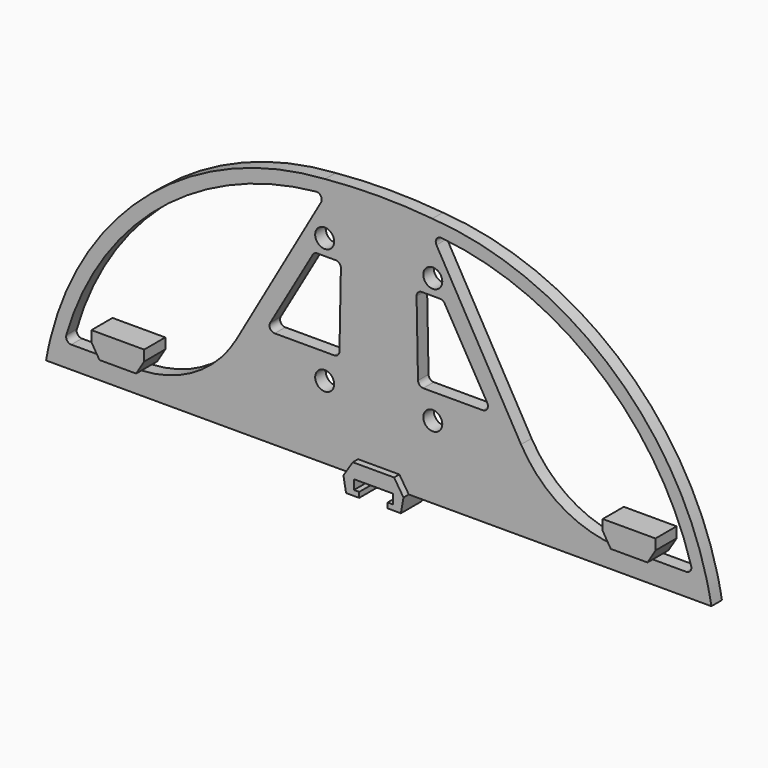
from build123d import *

# Parameters (mm, degrees)
F0_R     = 18
F1_DEPTH = 12.5
F2_R     = 10
F3_DEPTH = 25


# Not quite as in the source:
# - a feature names something its author has since deleted; it is built from what else it names


with BuildPart() as f1:
    # F0 (on Front) → F1 (new body, symmetric)
    with BuildSketch(Plane.XZ):
        with BuildLine():
            Line((56.9371554598, -75), (595.9911190147, -75))
            Line((595.9911190147, -75), (595.9911190147, -33))
            Line((595.9911190147, -33), (519.5849960263, -33))
            Line((519.5849960263, -33), (450, -33))
            ThreePointArc((450, -33), (345.7777045638, -0.7457623443), (269.8662378191, 77.6128487294))
            Line((269.8662378191, 77.6128487294), (100, 375))
            Line((100, 375), (0, 375))
            Line((0, 375), (-100, 375))
            Line((-100, 375), (-269.8662378191, 77.6128487294))
            ThreePointArc((-269.8662378191, 77.6128487294), (-345.7777045638, -0.7457623443), (-450, -33))
            Line((-450, -33), (-484.7924980132, -33))
            Line((-484.7924980132, -33), (-519.5849960263, -33))
            Line((-519.5849960263, -33), (-595.9911190147, -33))
            Line((-595.9911190147, -33), (-595.9911190147, -75))
            Line((-595.9911190147, -75), (-56.9371554598, -75))
            Line((-56.9371554598, -75), (-39.1645557923, -47.3871512706))
            Line((-39.1645557923, -47.3871512706), (3.3388429378, -47.3871512706))
            Line((3.3388429378, -47.3871512706), (39.1645557923, -47.3871512706))
            Line((39.1645557923, -47.3871512706), (56.9371554598, -75))
        make_face()
        with Locations((-102.5, 63)):
            Circle(F0_R, mode=Mode.SUBTRACT)
        with Locations((102.5, 63)):
            Circle(F0_R, mode=Mode.SUBTRACT)
        with BuildLine():
            ThreePointArc((-74.4771999255, 121.0282629209), (-77.4732139948, 114.0830094681), (-84.4753157308, 111.2223771768))
            Line((-84.4753157308, 111.2223771768), (-197.1059338565, 111.2223771768))
            ThreePointArc((-197.1059338565, 111.2223771768), (-205.7661878943, 116.2223771768), (-205.7661878943, 126.2223771768))
            Line((-205.7661878943, 126.2223771768), (-125.0655397306, 266))
            ThreePointArc((-125.0655397306, 266), (-121.4052856928, 269.6602540378), (-116.4052856928, 271))
            Line((-116.4052856928, 271), (-81.7615214746, 271))
            ThreePointArc((-81.7615214746, 271), (-74.622153766, 268.0021017359), (-71.7634056693, 260.8058857441))
            Line((-71.7634056693, 260.8058857441), (-74.4771999255, 121.0282629209))
        make_face(mode=Mode.SUBTRACT)
        with Locations((-102.5, 301)):
            Circle(F0_R, mode=Mode.SUBTRACT)
        with BuildLine():
            ThreePointArc((84.4753157308, 111.2223771768), (77.4732139948, 114.0830094681), (74.4771999255, 121.0282629209))
            Line((74.4771999255, 121.0282629209), (71.7634056693, 260.8058857441))
            ThreePointArc((71.7634056693, 260.8058857441), (74.622153766, 268.0021017359), (81.7615214746, 271))
            Line((81.7615214746, 271), (116.4052856928, 271))
            ThreePointArc((116.4052856928, 271), (121.4052856928, 269.6602540378), (125.0655397306, 266))
            Line((125.0655397306, 266), (205.7661878943, 126.2223771768))
            ThreePointArc((205.7661878943, 126.2223771768), (205.7661878943, 116.2223771768), (197.1059338565, 111.2223771768))
            Line((197.1059338565, 111.2223771768), (84.4753157308, 111.2223771768))
        make_face(mode=Mode.SUBTRACT)
        with Locations((102.5, 301)):
            Circle(F0_R, mode=Mode.SUBTRACT)
        with BuildLine():
            ThreePointArc((100, 375), (413.732568712, 250.914148912), (595.9911190147, -33))
            Line((595.9911190147, -33), (621.814123166, -33))
            ThreePointArc((621.814123166, -33), (432.1619331745, 268.1134366241), (101.6213617791, 399.9473683177))
            ThreePointArc((101.6213617791, 399.9473683177), (0, 404.6514727579), (-101.6213617791, 399.9473683177))
            ThreePointArc((-101.6213617791, 399.9473683177), (-432.1619331745, 268.1134366241), (-621.814123166, -33))
            Line((-621.814123166, -33), (-595.9911190147, -33))
            ThreePointArc((-595.9911190147, -33), (-413.732568712, 250.914148912), (-100, 375))
            Line((-100, 375), (0, 375))
            Line((0, 375), (100, 375))
        make_face()
        with BuildLine():
            Line((-595.9911190147, -75), (-595.9911190147, -33))
            Line((-595.9911190147, -33), (-621.814123166, -33))
            ThreePointArc((-621.814123166, -33), (-626.6847460238, -53.9163527136), (-630.7708927375, -75))
            Line((-630.7708927375, -75), (-595.9911190147, -75))
        make_face()
        with BuildLine():
            Line((595.9911190147, -33), (595.9911190147, -75))
            Line((595.9911190147, -75), (630.7708927375, -75))
            ThreePointArc((630.7708927375, -75), (626.6847460238, -53.9163527136), (621.814123166, -33))
            Line((621.814123166, -33), (595.9911190147, -33))
        make_face()
    extrude(amount=F1_DEPTH, both=True)

    # F2
    f2_edges = [f1.edges().sort_by_distance(p)[0] for p in [
        (-100, 0, 375),
        (100, 0, 375),
        (595.991119, 0, -33),
        (-595.991119, 0, -33),
    ]]
    fillet(f2_edges, radius=F2_R)

    # F0 (on Front) → F3 (join, symmetric)
    with BuildSketch(Plane.XZ):
        Polygon((-484.7924980132, -33), (-450, -33), (-434.7924980132, -8), (-434.7924980132, 12), (-484.7924980132, 12), (-534.7924980132, 12), (-534.7924980132, -8), (-519.5849960263, -33), align=None)
        Polygon((37, -75), (56.9371554598, -75), (39.1645557923, -47.3871512706), (3.3388429378, -47.3871512706), (-39.1645557923, -47.3871512706), (-56.9371554598, -75), (-37, -75), (0, -75), align=None)
        Polygon((52, -103), (56.9371554598, -75), (37, -75), (37, -93), (27, -93), (27, -103), align=None)
        Polygon((-37, -93), (-37, -75), (-56.9371554598, -75), (-52, -103), (-27, -103), (-27, -93), align=None)
        Polygon((450, -33), (519.5849960263, -33), (534.7924980132, -8), (534.7924980132, 12), (484.7924980132, 12), (434.7924980132, 12), (434.7924980132, -8), align=None)
    extrude(amount=F3_DEPTH, both=True)


solid = f1.part
